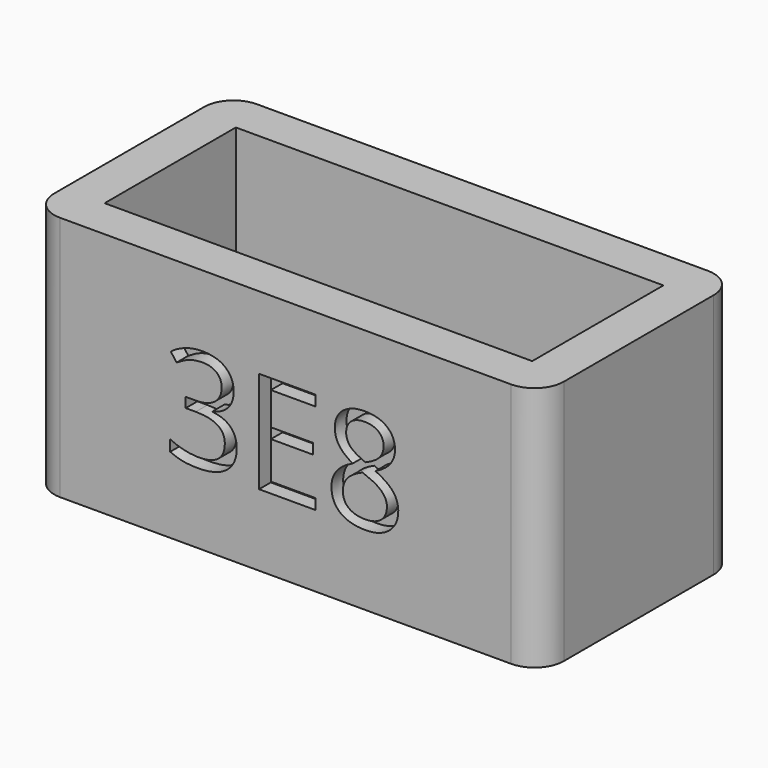
from build123d import *

# Parameters (mm, degrees)
F2_W         = 17.4
F2_H         = 8.4
F3_DEPTH     = 8.4
F4_W         = 14.6
F4_H         = 5.6
F5_DEPTH     = 7
F6_TEXT_SIZE = 4.8611111111
F7_DEPTH     = 0.5
F8_R         = 1


# Not quite as in the source:
# - Text() gives the source's letters only with a copy of the font that has no kerning and outlines rounded to 1/6400 em; it was checked with that copy


with BuildPart() as f3:
    # F2 (on Top) → F3 (new body)
    with BuildSketch(Plane.XY):
        Rectangle(F2_W, F2_H)
    extrude(amount=F3_DEPTH)

    # F4 (on face) → F5 (cut)
    with BuildSketch(Plane.XY.offset(8.4)):
        Rectangle(F4_W, F4_H)
    extrude(amount=-F5_DEPTH, mode=Mode.SUBTRACT)

    # F6 (on face) → F7 (cut)
    with BuildSketch(Plane.XZ.offset(4.2)):
        with Locations((-4.1627061632, 2.45)):
            Text('3E8', F6_TEXT_SIZE, font='Open Sans', text_align=(TextAlign.LEFT, TextAlign.BOTTOM))
    extrude(amount=-F7_DEPTH, mode=Mode.SUBTRACT)

    # F8
    f8_edges = [f3.edges().sort_by_distance(p)[0] for p in [
        (8.7, -4.2, 4.2),
        (8.7, 4.2, 4.2),
        (-8.7, 4.2, 4.2),
        (-8.7, -4.2, 4.2),
    ]]
    fillet(f8_edges, radius=F8_R)


solid = f3.part
